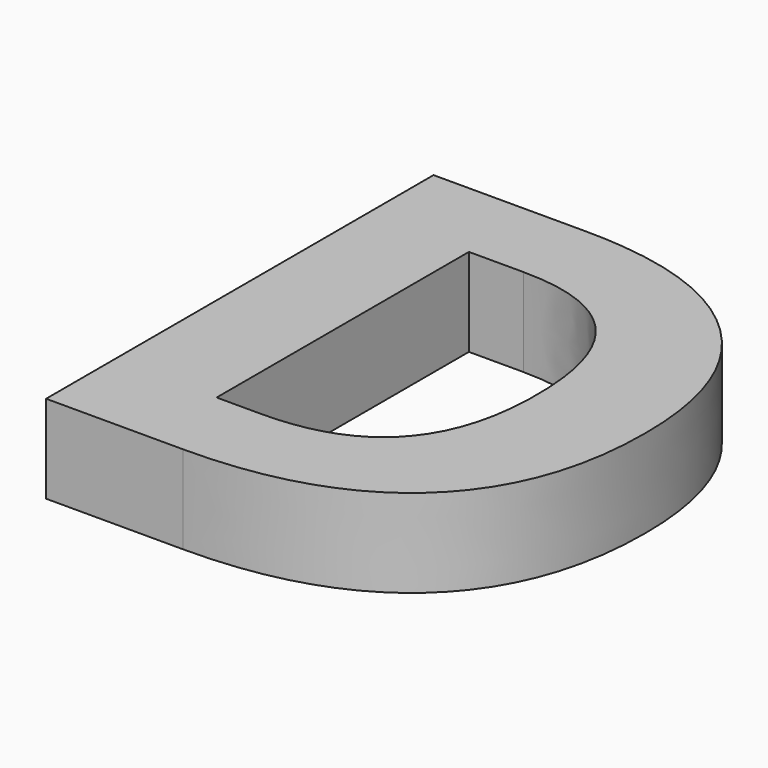
from build123d import *

# Parameters (mm, degrees)
F0_TEXT_SIZE = 77.0596580373
F1_DEPTH     = 10


# Not quite as in the source:
# - Text() gives the source's letters only with a copy of the font that has no kerning and outlines rounded to 1/6400 em; it was checked with that copy


with BuildPart() as f1:
    # F0 (on Top) → F1 (new body)
    with BuildSketch(Plane.XY):
        with Locations((0, 0)):
            Text('D', F0_TEXT_SIZE, font='Open Sans', font_style=FontStyle.BOLD, text_align=(TextAlign.LEFT, TextAlign.BOTTOM))
    extrude(amount=F1_DEPTH)


solid = f1.part
